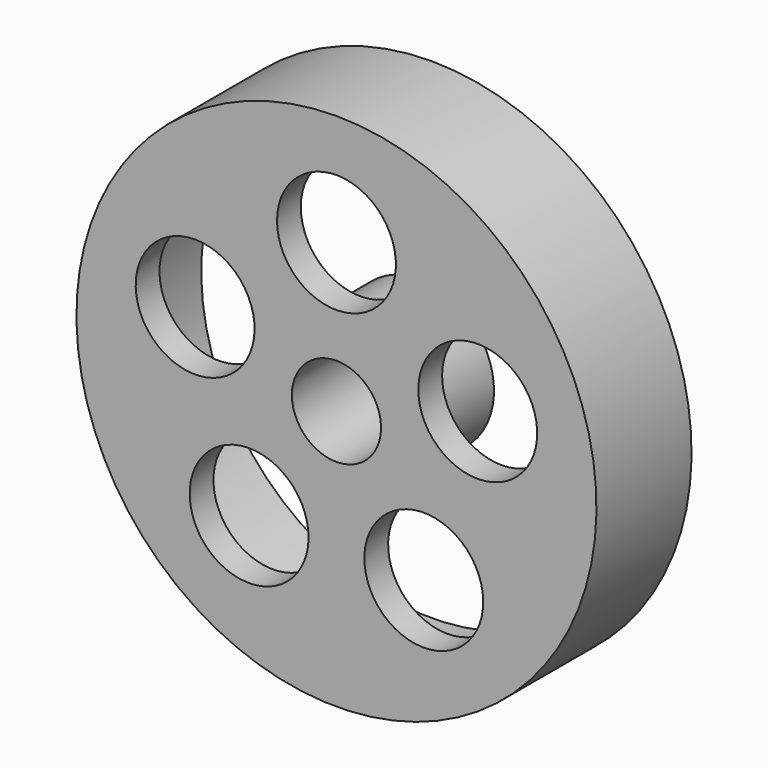
from build123d import *

# Parameters (mm, degrees)
F0_W            = 8
F0_H            = 17.5
F3_D            = 6
F4_T            = -2
F6_D            = 8
F6_COPIES_COUNT = 5
F7_SIZE         = 1


# Not quite as in the source:
# - a pattern or mirror of a feature is missing from the dataset's text; its kind, count and spacing are read off the source's solid


with BuildPart() as f1:
    # F0 (on Right) → F1 (revolve)
    with BuildSketch(Plane.YZ):
        with Locations((4, 8.75)):
            Rectangle(F0_W, F0_H)
    revolve(axis=Axis((0, 4, 0), (0, 1, 0)))

    # F3 (through all)
    with Locations(Plane.XZ):
        with Locations((0, 0)):
            Hole(F3_D / 2)

    # F4
    f4_openings = [f1.faces().sort_by_distance(p)[0] for p in [
        (0, 8, -17.005025),
    ]]
    offset(amount=F4_T, openings=f4_openings)

    # F6 (through all)
    with Locations(Plane.XZ):
        with Locations((0, 10)):
            f6 = Hole(F6_D / 2)

    # F6_copies: F6 ×5 about axis
    f6_copies_axis = Axis((0, 0, 0), (0, 1, 0))
    for i in range(1, F6_COPIES_COUNT):
        add(f6.rotate(f6_copies_axis, i * 360 / F6_COPIES_COUNT), mode=Mode.SUBTRACT)

    # F7
    f7_edges = [f1.edges().sort_by_distance(p)[0] for p in [
        (-5, 8, 0),
    ]]
    chamfer(f7_edges, length=F7_SIZE)


solid = f1.part
